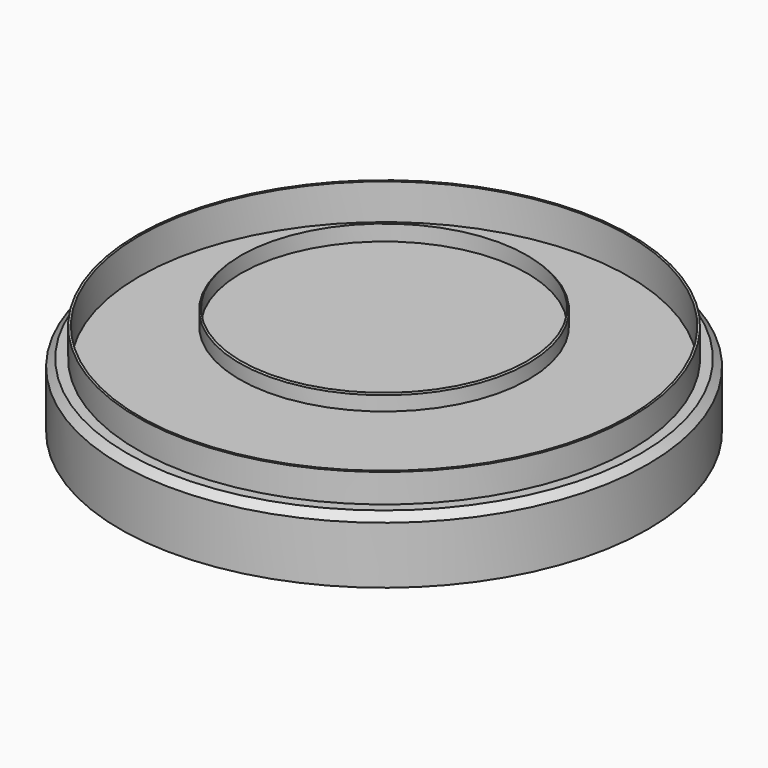
from build123d import *

# Parameters (mm, degrees)
F0_R      = 9.225
F1_DEPTH  = 2.25
F2_R      = 8.625
F3_DEPTH  = 1
F4_DEPTH  = 1
F5_R      = 5.05
F6_DEPTH  = 0.75
F7_R      = 5
F8_DEPTH  = 0.75
F10_R     = 8.55
F11_DEPTH = 1.25
F12_R     = 7.5
F13_DEPTH = 1
F14_SIZE  = 0.25


# Not quite as in the source:
# - a fillet or chamfer that OpenCascade refuses, or shapes differently, is made with other operations: its cross-section is extruded or revolved along the edge and cut away or added


with BuildPart() as f1:
    # F0 (on Top) → F1 (new body)
    with BuildSketch(Plane.XY):
        Circle(F0_R)
    extrude(amount=F1_DEPTH)

    # F2 (on face) → F3 (join)
    with BuildSketch(Plane.XY.offset(2.25)):
        Circle(F2_R)
    extrude(amount=F3_DEPTH)

    # F2 (on face) → F4 (join)
    with BuildSketch(Plane.XY.offset(2.25)):
        Circle(F2_R)
    extrude(amount=F4_DEPTH)

    # F5 (on face) → F6 (join)
    with BuildSketch(Plane.XY.offset(3.25)):
        Circle(F5_R)
    extrude(amount=F6_DEPTH)

    # F7 (on face) → F8 (cut)
    with BuildSketch(Plane.XY.offset(4)):
        Circle(F7_R)
    extrude(amount=-F8_DEPTH, mode=Mode.SUBTRACT)

    # F10 (on offset) → F11 (cut)
    with BuildSketch(Plane.XY.offset(3.25)):
        Circle(F10_R)
    extrude(amount=-F11_DEPTH, mode=Mode.SUBTRACT)

    # F12 (on face) → F13 (cut)
    with BuildSketch(Plane(origin=(0, 0, 0), x_dir=(1, 0, 0), z_dir=(0, 0, -1))):
        Circle(F12_R)
    extrude(amount=-F13_DEPTH, mode=Mode.SUBTRACT)

    # F14
    f14_edges = [f1.edges().sort_by_distance(p)[0] for p in [
        (-7.5, 0, 1),
    ]]
    chamfer(f14_edges, length=F14_SIZE)

    # F15: chamfer of 0.25 on 1 edges, made by hand

    # F15_s1 → F15_t2 (revolve, cut)
    with BuildSketch(Plane.XZ):
        Polygon((9.225, 2), (8.975, 2.25), (9.225, 2.25), align=None)
    revolve(axis=Axis((0, 0, 2.25), (0, 0, 1)), mode=Mode.SUBTRACT)

    # F15#s1: chamfer of 0.25 on 1 edges, made by hand

    # F15_s1_s1 → F15_s1_t2 (revolve, cut)
    with BuildSketch(Plane.XZ):
        Polygon((5.05, 3.75), (4.8, 4), (5.05, 4), align=None)
    revolve(axis=Axis((0, 0, 4), (0, 0, 1)), mode=Mode.SUBTRACT)


solid = f1.part
